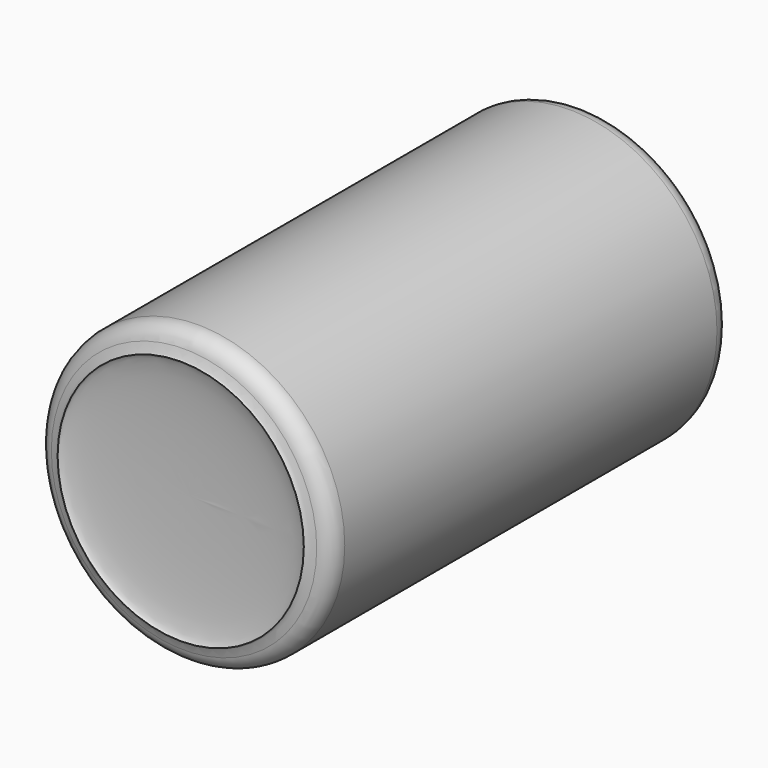
from build123d import *

# Parameters (mm, degrees)
F3_DEPTH = 0.0254


with BuildPart() as f1:
    # F0 (on Top) → F1 (revolve)
    with BuildSketch(Plane.XY):
        with BuildLine():
            Line((6.5402514301, 69.8725463986), (6.5402514301, 1.6435814323))
            add(Edge.make_bspline(
                [(6.5402514301, 1.6435814323), (16.6055685907, 1.6237888089), (24.4864700581, 1.0951121643), (24.2117271912, 0)],
                knots=[0, 0, 0, 0, 0.7582969465, 0.7582969465, 0.7582969465, 0.7582969465], degree=3))
            add(Edge.make_bspline(
                [(25.5896002368, 0.5953258758), (24.9631976139, 0.4681905354), (24.4171222, 0.2947845137), (24.2117271912, 0)],
                knots=[0.3083695275, 0.3083695275, 0.3083695275, 0.3083695275, 0.5848021934, 0.5848021934, 0.5848021934, 0.5848021934], degree=3))
            ThreePointArc((25.5896002368, 0.5953258758), (27.050958138, 1.47703779), (27.624379952, 3.0845732447))
            Line((27.624379952, 3.0845732447), (27.624379952, 69.8725463986))
            ThreePointArc((27.624379952, 69.8725463986), (26.8804311762, 71.6685976229), (25.084379952, 72.4125463986))
            add(Edge.make_bspline(
                [(25.084379952, 72.4125463986), (24.711275029, 71.678932761), (24.5228062968, 70.0934224878), (23.9885225892, 69.8725463986)],
                knots=[0, 0, 0, 0, 0.3680062222, 0.3680062222, 0.3680062222, 0.3680062222], degree=3))
            add(Edge.make_bspline(
                [(23.9885225892, 69.8725463986), (23.8915327068, 69.8324501995), (23.783146815, 69.837324245), (23.6659098082, 69.8725463986)],
                knots=[0.3680062222, 0.3680062222, 0.3680062222, 0.3680062222, 0.4348113291, 0.4348113291, 0.4348113291, 0.4348113291], degree=3))
            Line((23.6659098082, 69.8725463986), (6.5402514301, 69.8725463986))
        make_face()
        with BuildLine():
            Line((23.9885225892, 69.8725463986), (23.6659098082, 69.8725463986))
            add(Edge.make_bspline(
                [(23.9885225892, 69.8725463986), (23.8915327068, 69.8324501995), (23.783146815, 69.837324245), (23.6659098082, 69.8725463986)],
                knots=[0.3680062222, 0.3680062222, 0.3680062222, 0.3680062222, 0.4348113291, 0.4348113291, 0.4348113291, 0.4348113291], degree=3))
        make_face()
    revolve(axis=Axis((6.5402514301, 35.7580639155, 0), (0, 1, 0)))

    # F2 (on face) → F3 (join)
    with BuildSketch(Plane(origin=(0, 69.8725463986, 0), x_dir=(-1, 0, 0), z_dir=(0, 1, 0))):
        with BuildLine():
            ThreePointArc((-3.4999095369, 12.8522840624), (-3.3524060249, 13.5768925878), (-3.4999095369, 14.3015011132))
            ThreePointArc((-3.4999095369, 14.3015011132), (-6.7963991448, 16.4044588849), (-10.0287375972, 14.2041718005))
            ThreePointArc((-10.0287375972, 14.2041718005), (-10.1516131859, 13.5282279315), (-10.0287375972, 12.8522840624))
            ThreePointArc((-10.0287375972, 12.8522840624), (-6.764323567, 12.3472555866), (-3.4999095369, 12.8522840624))
        make_face()
    extrude(amount=F3_DEPTH)


solid = f1.part
